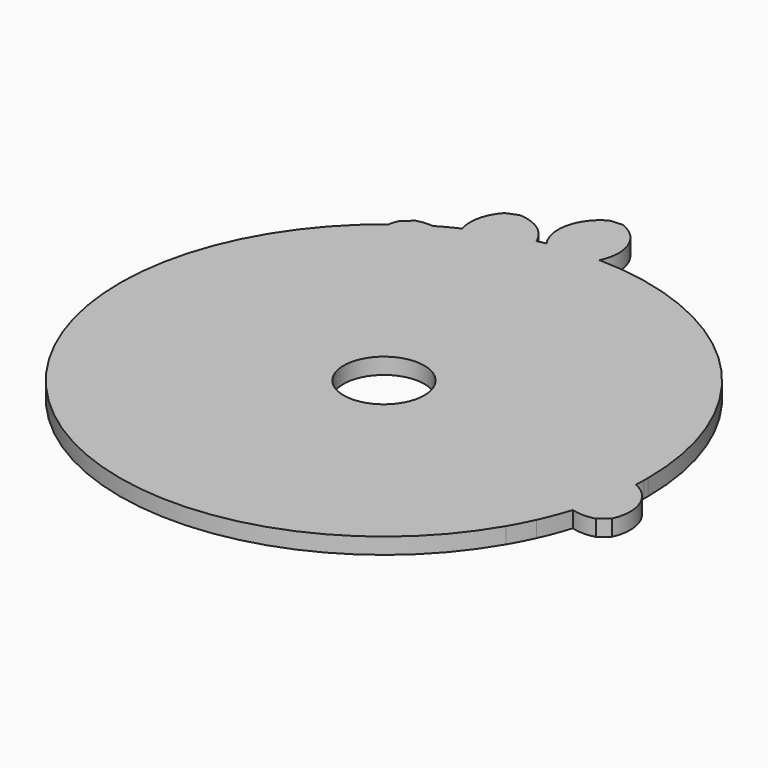
from build123d import *

# Parameters (mm, degrees)
F1_R     = 2.5
F2_DEPTH = 1


with BuildPart() as f2:
    # F1 (on Top) → F2 (new body)
    with BuildSketch(Plane.XY):
        with BuildLine():
            ThreePointArc((-2.8225697973, 16.1183651398), (-1.2838761119, 16.3131927338), (0.2663514513, 16.3614685143))
            ThreePointArc((0.2663514513, 16.3614685143), (0.3425890016, 18.4864230236), (-1.1856698611, 19.9648237403))
            Line((-1.1856698611, 19.9648237403), (-1.9521142238, 19.9045032607))
            ThreePointArc((-1.9521142238, 19.9045032607), (-3.2302848587, 18.2052317525), (-2.8225697973, 16.1183651398))
        make_face()
        with BuildLine():
            ThreePointArc((16.360600111, -0.3152127039), (16.3628772829, -0.1576136634), (16.3636363636, 0))
            ThreePointArc((16.3636363636, 0), (11.6646275838, 11.4762824283), (0.2663514513, 16.3614685143))
            ThreePointArc((0.2663514513, 16.3614685143), (-1.2838761119, 16.3131927338), (-2.8225697973, 16.1183651398))
            ThreePointArc((-2.8225697973, 16.1183651398), (-3.0952881484, 16.0682228737), (-3.3671176898, 16.0134666298))
            ThreePointArc((-3.3671176898, 16.0134666298), (-5.2140285038, 15.5107221561), (-6.9895966639, 14.7957471429))
            ThreePointArc((-6.9895966639, 14.7957471429), (-7.637404231, 14.4719954275), (-8.2702526578, 14.1198978756))
            ThreePointArc((-8.2702526578, 14.1198978756), (-9.1779617865, 13.5474577869), (-10.0461981882, 12.9167525719))
            ThreePointArc((-10.0461981882, 12.9167525719), (-10.7718419373, -12.3181174016), (14.1409449401, -8.2342134562))
            ThreePointArc((14.1409449401, -8.2342134562), (14.5297243379, -7.5269984527), (14.8831626027, -6.8014752798))
            ThreePointArc((14.8831626027, -6.8014752798), (15.2794397939, -5.8572446275), (15.6158812541, -4.8900764513))
            ThreePointArc((15.6158812541, -4.8900764513), (16.1012982128, -2.9183541432), (16.3387742935, -0.9016926457))
            ThreePointArc((16.3387742935, -0.9016926457), (16.352316695, -0.6085505312), (16.360600111, -0.3152127039))
        make_face()
        Circle(F1_R, mode=Mode.SUBTRACT)
        with BuildLine():
            ThreePointArc((-6.9895966639, 14.7957471429), (-5.2140285038, 15.5107221561), (-3.3671176898, 16.0134666298))
            ThreePointArc((-3.3671176898, 16.0134666298), (-4.2906994467, 17.1695948436), (-5.6940409736, 17.6389223059))
            Line((-5.6940409736, 17.6389223059), (-6.4043328259, 17.3447097874))
            ThreePointArc((-6.4043328259, 17.3447097874), (-7.0387105861, 16.1486962619), (-6.9895966639, 14.7957471429))
        make_face()
        with BuildLine():
            ThreePointArc((-10.0461981882, 12.9167525719), (-9.1779617865, 13.5474577869), (-8.2702526578, 14.1198978756))
            ThreePointArc((-8.2702526578, 14.1198978756), (-8.7707794497, 14.1245479657), (-9.2630136276, 14.0336952997))
            Line((-9.2630136276, 14.0336952997), (-9.847624654, 13.5343903136))
            ThreePointArc((-9.847624654, 13.5343903136), (-9.9661500626, 13.2317567594), (-10.0461981882, 12.9167525719))
        make_face()
        with BuildLine():
            ThreePointArc((17.6530775237, -4.3953792078), (17.7296643017, -2.3725080911), (16.3387742935, -0.9016926457))
            ThreePointArc((16.3387742935, -0.9016926457), (16.1012982128, -2.9183541432), (15.6158812541, -4.8900764513))
            ThreePointArc((15.6158812541, -4.8900764513), (16.3418473368, -4.9953212922), (17.0684664973, -4.894684194))
            Line((17.0684664973, -4.894684194), (17.6530775237, -4.3953792078))
        make_face()
    extrude(amount=F2_DEPTH)


solid = f2.part
